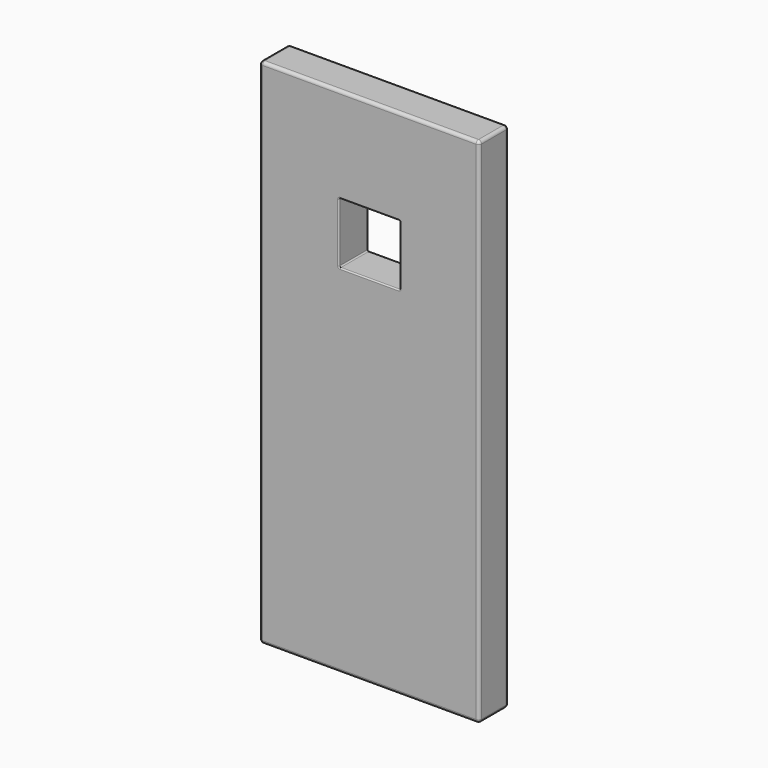
from build123d import *

# Parameters (mm, degrees)
F0_W     = 914.4
F0_H     = 2133.6
F1_DEPTH = 152.4
F2_R     = 12.7
F3_R     = 5.08


# Not quite as in the source:
# - a feature names something its author has since deleted; it is built from what else it names


with BuildPart() as f1:
    # F0 (on Front) → F1 (new body)
    with BuildSketch(Plane.XZ):
        with Locations((457.2, 1066.8)):
            Rectangle(F0_W, F0_H)
        Polygon((330.2, 1737.36), (457.2, 1737.36), (584.2, 1737.36), (584.2, 1483.36), (330.2, 1483.36), align=None, mode=Mode.SUBTRACT)
    extrude(amount=F1_DEPTH)

    # F2
    f2_edges = [f1.edges().sort_by_distance(p)[0] for p in [
        (457.2, -152.4, 2133.6),
        (914.4, -152.4, 1066.8),
        (914.4, -76.2, 2133.6),
        (457.2, 0, 2133.6),
        (914.4, 0, 1066.8),
        (914.4, -76.2, 0),
        (457.2, -152.4, 0),
        (0, -152.4, 1066.8),
        (457.2, 0, 0),
        (0, 0, 1066.8),
        (0, -76.2, 0),
        (0, -76.2, 2133.6),
    ]]
    fillet(f2_edges, radius=F2_R)

    # F3
    f3_edges = [f1.edges().sort_by_distance(p)[0] for p in [
        (457.2, -152.4, 1483.36),
        (330.2, -152.4, 1610.36),
        (457.2, -152.4, 1737.36),
        (457.2, 0, 1483.36),
        (330.2, 0, 1610.36),
        (584.2, 0, 1610.36),
        (457.2, 0, 1737.36),
        (584.2, -152.4, 1610.36),
        (584.2, -76.2, 1483.36),
        (330.2, -76.2, 1483.36),
        (330.2, -76.2, 1737.36),
        (584.2, -76.2, 1737.36),
    ]]
    fillet(f3_edges, radius=F3_R)


solid = f1.part
